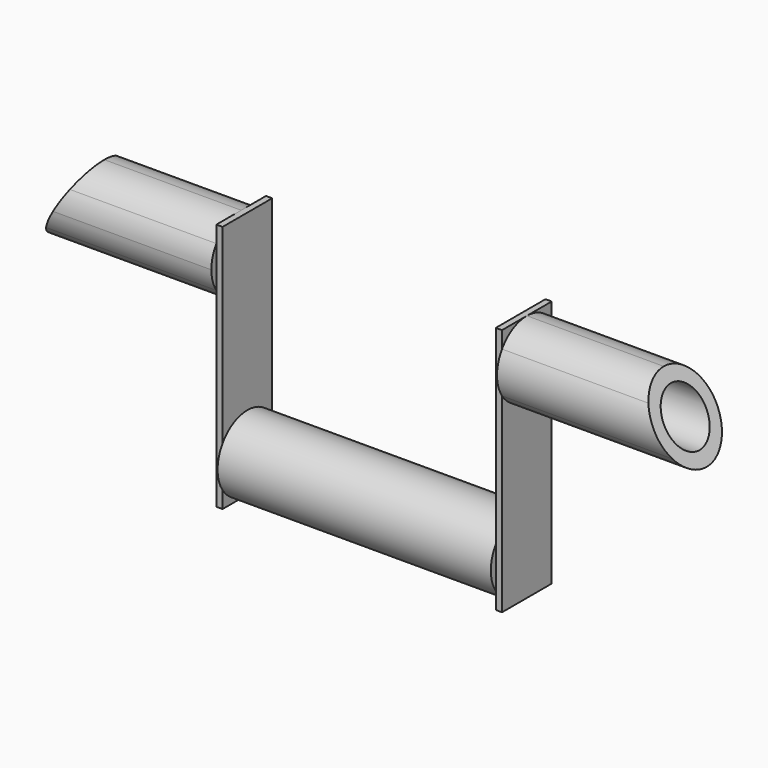
from build123d import *

# Parameters (mm, degrees)
F0_R         = 19.05
F0_R_2       = 12.7
F2_DEPTH     = 69.85
F3_W         = 31.75
F3_H         = 127
F4_DEPTH     = 3.175
F5_R         = 12.7
F6_DEPTH     = 101.6
F7_R         = 12.7
F8_DEPTH     = 3.175
F9_R         = 12.7
F10_DEPTH    = 101.6
F6_FACE_R    = 19.05
F6_FACE_R_2  = 12.7
F13_REACH    = 74.5272199335
F10_FACE_R   = 19.05
F10_FACE_R_2 = 12.7
F14_REACH    = 74.5272199335


with BuildPart() as f2:
    # F0 (on Right) → F2 (new body, symmetric)
    with BuildSketch(Plane.YZ):
        Circle(F0_R)
        Circle(F0_R_2, mode=Mode.SUBTRACT)
    extrude(amount=F2_DEPTH, both=True)

    # F3 (on face) → F4 (join)
    with BuildSketch(Plane.YZ.offset(69.85)):
        with Locations((0, 44.45)):
            Rectangle(F3_W, F3_H)
    extrude(amount=F4_DEPTH)

    # F5 (on face) → F6 (join)
    with BuildSketch(Plane.YZ.offset(73.025)):
        with BuildLine():
            Line((15.875, 78.3697162906), (15.875, 99.4302837094))
            ThreePointArc((15.875, 99.4302837094), (9.0083459795, 105.6854759454), (-4.82e-08, 107.95))
            ThreePointArc((-4.82e-08, 107.95), (-9.0083460219, 105.6854759226), (-15.875, 99.4302837094))
            Line((-15.875, 99.4302837094), (-15.875, 78.3697162906))
            ThreePointArc((-15.875, 78.3697162906), (0, 69.85), (15.875, 78.3697162906))
        make_face()
        with Locations((0, 88.9)):
            Circle(F5_R, mode=Mode.SUBTRACT)
        with BuildLine():
            ThreePointArc((-15.875, 99.4302837094), (-19.05, 88.9), (-15.875, 78.3697162906))
            Line((-15.875, 78.3697162906), (-15.875, 99.4302837094))
        make_face()
        with BuildLine():
            ThreePointArc((15.875, 78.3697162906), (18.2389864028, 83.400738686), (19.05, 88.9))
            ThreePointArc((19.05, 88.9), (18.2389864028, 94.399261314), (15.875, 99.4302837094))
            Line((15.875, 99.4302837094), (15.875, 78.3697162906))
        make_face()
    extrude(amount=F6_DEPTH)

    # F7 (on face) → F8 (join)
    with BuildSketch(Plane(origin=(-69.85, 0, 0), x_dir=(0, -1, 0), z_dir=(-1, 0, 0))):
        with BuildLine():
            ThreePointArc((-15.875, 10.5302837094), (0, 19.05), (15.875, 10.5302837094))
            Line((15.875, 10.5302837094), (15.875, 107.95))
            Line((15.875, 107.95), (-15.875, 107.95))
            Line((-15.875, 107.95), (-15.875, 10.5302837094))
        make_face()
        with BuildLine():
            ThreePointArc((-15.875, -10.5302837094), (-9.0083460007, -16.785475934), (0, -19.05))
            ThreePointArc((0, -19.05), (9.0083460007, -16.785475934), (15.875, -10.5302837094))
            Line((15.875, -10.5302837094), (15.875, 10.5302837094))
            ThreePointArc((15.875, 10.5302837094), (0, 19.05), (-15.875, 10.5302837094))
            Line((-15.875, 10.5302837094), (-15.875, -10.5302837094))
        make_face()
        Circle(F7_R, mode=Mode.SUBTRACT)
        Circle(F7_R)
        with BuildLine():
            Line((0, -19.05), (15.875, -19.05))
            Line((15.875, -19.05), (15.875, -10.5302837094))
            ThreePointArc((15.875, -10.5302837094), (9.0083460007, -16.785475934), (0, -19.05))
        make_face()
        with BuildLine():
            Line((-15.875, -19.05), (0, -19.05))
            ThreePointArc((0, -19.05), (-9.0083460007, -16.785475934), (-15.875, -10.5302837094))
            Line((-15.875, -10.5302837094), (-15.875, -19.05))
        make_face()
    extrude(amount=F8_DEPTH)

    # F9 (on face) → F10 (join)
    with BuildSketch(Plane(origin=(-73.025, 0, 0), x_dir=(0, -1, 0), z_dir=(-1, 0, 0))):
        with BuildLine():
            Line((15.875, 78.3697162906), (15.875, 99.4302837094))
            ThreePointArc((15.875, 99.4302837094), (9.0083459795, 105.6854759454), (-4.82e-08, 107.95))
            ThreePointArc((-4.82e-08, 107.95), (-9.0083460219, 105.6854759226), (-15.875, 99.4302837094))
            Line((-15.875, 99.4302837094), (-15.875, 78.3697162906))
            ThreePointArc((-15.875, 78.3697162906), (0, 69.85), (15.875, 78.3697162906))
        make_face()
        with Locations((0, 88.9)):
            Circle(F9_R, mode=Mode.SUBTRACT)
        with BuildLine():
            ThreePointArc((15.875, 78.3697162906), (18.2389864028, 83.400738686), (19.05, 88.9))
            ThreePointArc((19.05, 88.9), (18.2389864028, 94.399261314), (15.875, 99.4302837094))
            Line((15.875, 99.4302837094), (15.875, 78.3697162906))
        make_face()
        with BuildLine():
            ThreePointArc((-15.875, 99.4302837094), (-19.05, 88.9), (-15.875, 78.3697162906))
            Line((-15.875, 78.3697162906), (-15.875, 99.4302837094))
        make_face()
    extrude(amount=F10_DEPTH)

    f13_end = Plane(origin=(153.9793167929, 0, 88.9), x_dir=(0.5, 0, -0.8660254038), z_dir=(-0.8660254038, 0, -0.5))
    # F6_face (on face) → F13 (cut, up to a plane its end follows)
    with BuildSketch(Plane(origin=(174.625, 0, 88.9), x_dir=(0, 1, 0), z_dir=(1, 0, 0))):
        Circle(F6_FACE_R)
        Circle(F6_FACE_R_2, mode=Mode.SUBTRACT)
    f13_long = extrude(amount=-F13_REACH, mode=Mode.PRIVATE)
    add(split(f13_long, bisect_by=f13_end, keep=Keep.BOTTOM, mode=Mode.PRIVATE), mode=Mode.SUBTRACT)

    f14_end = Plane(origin=(-153.9793167929, 0, 88.9), x_dir=(-0.5, 0, -0.8660254038), z_dir=(-0.8660254038, 0, 0.5))
    # F10_face (on face) → F14 (cut, up to a plane its end follows)
    with BuildSketch(Plane(origin=(-174.625, 0, 88.9), x_dir=(0, -1, 0), z_dir=(-1, 0, 0))):
        Circle(F10_FACE_R)
        Circle(F10_FACE_R_2, mode=Mode.SUBTRACT)
    f14_long = extrude(amount=-F14_REACH, mode=Mode.PRIVATE)
    add(split(f14_long, bisect_by=f14_end, keep=Keep.TOP, mode=Mode.PRIVATE), mode=Mode.SUBTRACT)


solid = f2.part
